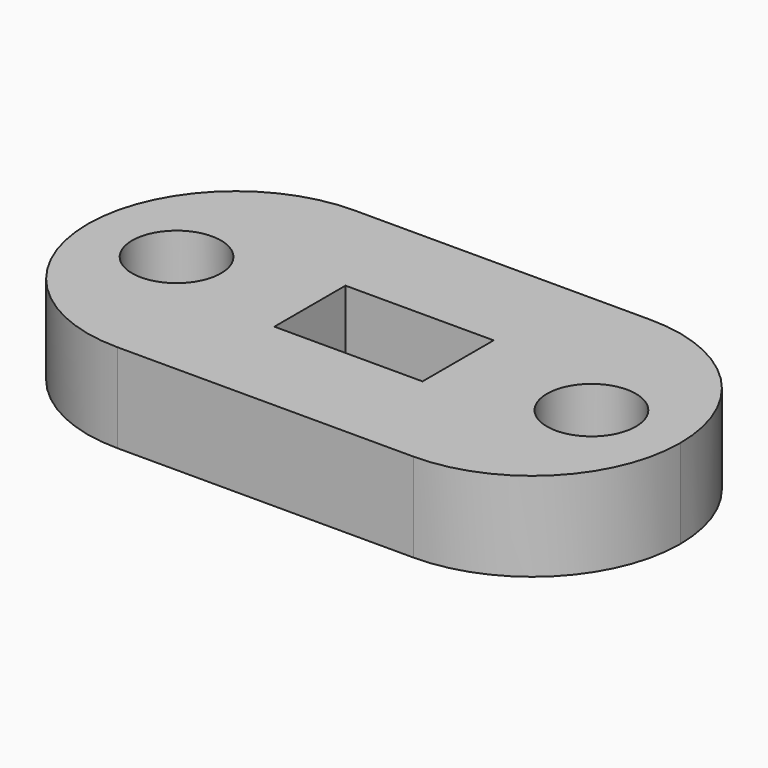
from build123d import *

# Parameters (mm, degrees)
F0_W     = 20
F0_H     = 10
F0_W_2   = 5
F0_H_2   = 3
F1_DEPTH = 3
F2_R     = 4.99999
F4_D     = 3


# Not quite as in the source:
# - a fillet or chamfer is up to 0.001 mm smaller than in the source, because OpenCascade refuses the exact size


with BuildPart() as f1:
    # F0 (on Top) → F1 (new body)
    with BuildSketch(Plane.XY):
        Rectangle(F0_W, F0_H)
        Rectangle(F0_W_2, F0_H_2, mode=Mode.SUBTRACT)
    extrude(amount=-F1_DEPTH)

    # F2 (radius 5 in the source; OpenCascade refuses exactly that, so slightly less here)
    f2_edges = [f1.edges().sort_by_distance(p)[0] for p in [
        (-10, -5, -1.5),
        (-10, 5, -1.5),
        (10, -5, -1.5),
        (10, 5, -1.5),
    ]]
    fillet(f2_edges, radius=F2_R)

    # F4 (through all)
    with Locations(Plane.XY):
        with Locations((-7, 0), (7, 0)):
            Hole(F4_D / 2)


solid = f1.part
